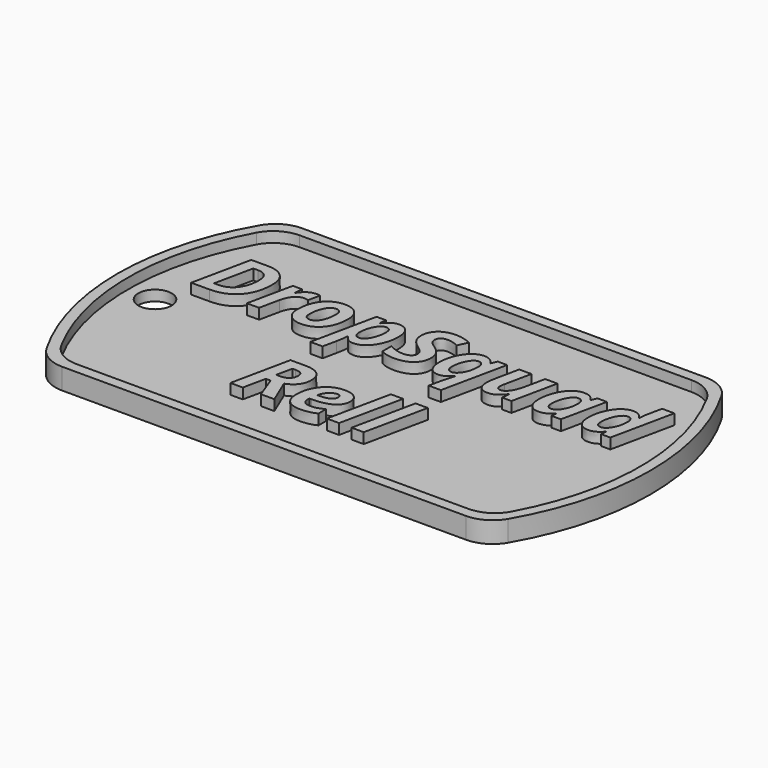
from build123d import *

# Parameters (mm, degrees)
F1_DEPTH     = 1
F3_DEPTH     = 1
F4_R         = 1.5875
F5_DEPTH     = 1
F6_TEXT_SIZE = 7.9327068912
F7_DEPTH     = 1


# Not quite as in the source:
# - Text() gives the source's letters only with a copy of the font that has no kerning and outlines rounded to 1/6400 em; it was checked with that copy


with BuildPart() as f1:
    # F0 (on Top) → F1 (new body)
    with BuildSketch(Plane.XY):
        with BuildLine():
            ThreePointArc((-19.2474145991, 14.2875), (-20.8349145991, 13.862130657), (-21.9970452561, 12.7))
            ThreePointArc((-21.9970452561, 12.7), (-25.4, 0), (-21.9970452561, -12.7))
            ThreePointArc((-21.9970452561, -12.7), (-20.8349145991, -13.862130657), (-19.2474145991, -14.2875))
            Line((-19.2474145991, -14.2875), (19.2474145991, -14.2875))
            ThreePointArc((19.2474145991, -14.2875), (20.8349145991, -13.862130657), (21.9970452561, -12.7))
            ThreePointArc((21.9970452561, -12.7), (25.4, 0), (21.9970452561, 12.7))
            ThreePointArc((21.9970452561, 12.7), (20.8349145991, 13.862130657), (19.2474145991, 14.2875))
            Line((19.2474145991, 14.2875), (-19.2474145991, 14.2875))
        make_face()
    extrude(amount=F1_DEPTH)

    # F2 (on face) → F3 (join)
    with BuildSketch(Plane.XY.offset(1)):
        with BuildLine():
            Line((19.2474145991, 14.2875), (-19.2474145991, 14.2875))
            ThreePointArc((-19.2474145991, 14.2875), (-20.8349145991, 13.862130657), (-21.9970452561, 12.7))
            ThreePointArc((-21.9970452561, 12.7), (-25.4, 0), (-21.9970452561, -12.7))
            ThreePointArc((-21.9970452561, -12.7), (-20.8349145991, -13.862130657), (-19.2474145991, -14.2875))
            Line((-19.2474145991, -14.2875), (19.2474145991, -14.2875))
            ThreePointArc((19.2474145991, -14.2875), (20.8349145991, -13.862130657), (21.9970452561, -12.7))
            ThreePointArc((21.9970452561, -12.7), (25.4, 0), (21.9970452561, 12.7))
            ThreePointArc((21.9970452561, 12.7), (20.8349145991, 13.862130657), (19.2474145991, 14.2875))
        make_face()
        with BuildLine():
            ThreePointArc((-21.4526124879, 11.6252061249), (-20.2856017842, 12.8404540819), (-18.6611352482, 13.2875))
            Line((-18.6611352482, 13.2875), (18.6611352482, 13.2875))
            ThreePointArc((18.6611352482, 13.2875), (20.2856017842, 12.8404540819), (21.4526124879, 11.6252061249))
            ThreePointArc((21.4526124879, 11.6252061249), (24.4, 0), (21.4526124879, -11.6252061249))
            ThreePointArc((21.4526124879, -11.6252061249), (20.2856017842, -12.8404540819), (18.6611352482, -13.2875))
            Line((18.6611352482, -13.2875), (-18.6611352482, -13.2875))
            ThreePointArc((-18.6611352482, -13.2875), (-20.2856017842, -12.8404540819), (-21.4526124879, -11.6252061249))
            ThreePointArc((-21.4526124879, -11.6252061249), (-24.4, 0), (-21.4526124879, 11.6252061249))
        make_face(mode=Mode.SUBTRACT)
    extrude(amount=F3_DEPTH)

    # F4 (on face) → F5 (cut)
    with BuildSketch(Plane.XY.offset(1)):
        with Locations((-21.821282804, 0)):
            Circle(F4_R)
    extrude(amount=-F5_DEPTH, mode=Mode.SUBTRACT)

    # F6 (on face) → F7 (join)
    with BuildSketch(Plane.XY.offset(1)):
        with Locations((-20.4074829817, 2.2829135123)):
            Text('DropSquad', F6_TEXT_SIZE, font='Open Sans', font_style=FontStyle.BOLDITALIC, text_align=(TextAlign.LEFT, TextAlign.BOTTOM))
        with Locations((-8.039897144, -8.5055678598)):
            Text('Rell', F6_TEXT_SIZE, font='Open Sans', font_style=FontStyle.BOLDITALIC, text_align=(TextAlign.LEFT, TextAlign.BOTTOM))
    extrude(amount=F7_DEPTH)


solid = f1.part
